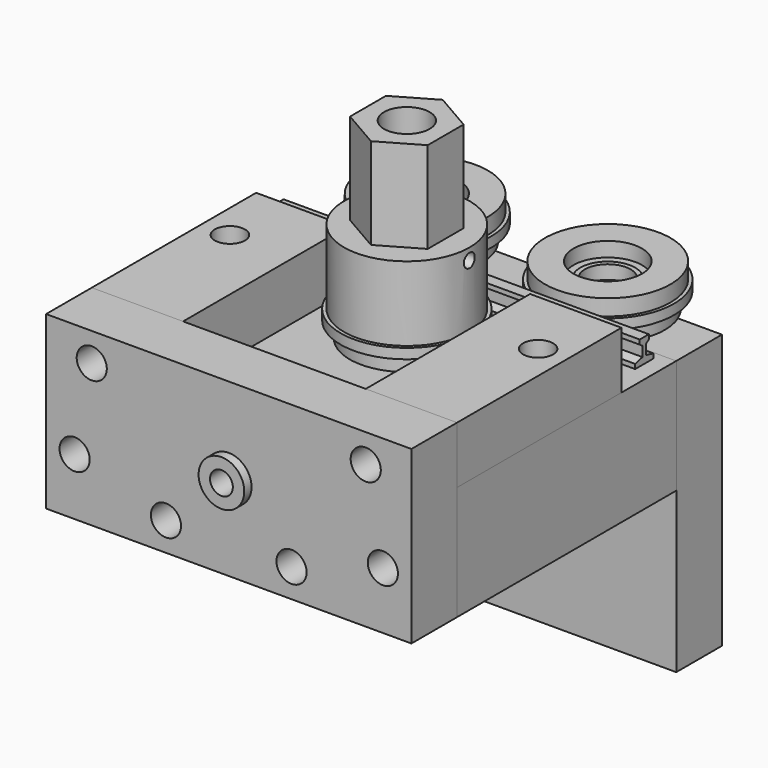
from build123d import *

# Parameters (mm, degrees)
F2_W           = 80
F2_H           = 12.5
F3_DEPTH       = 60
F6_DEPTH       = 40
F6_DEPTH_BACK  = 40
F4_W           = 2.5
F4_H           = 4
F12_R          = 7.5
F12_R_2        = 5
F13_DEPTH      = 20
F14_DEPTH      = 5
F17_R          = 3.3
F17_R_2        = 2.5
F18_DEPTH      = 60
F17_W          = 55
F17_H          = 12.5
F19_DEPTH      = 60
F21_DEPTH      = 12.5
F22_W          = 20
F22_H          = 45
F23_DEPTH      = 12.5
F24_W          = 80
F24_H          = 37.5
F25_DEPTH      = 12.5
F26_R          = 2.5
F27_DEPTH      = 25
F26_R_2        = 5
F26_R_3        = 3.3
F28_DEPTH      = 12.501
F29_R          = 2.5
F30_DEPTH      = 25
F29_R_2        = 3.3
F31_DEPTH      = 43.001
F32_DEPTH      = 20.751
F33_DEPTH      = 25
F34_R          = 4
F35_DEPTH      = 10
F37_DEPTH      = 14.5
F26_R_4        = 6
F38_DEPTH      = 2
F39_R          = 5
F39_R_2        = 2.5
F40_DEPTH      = 2
F41_DEPTH      = 2
F39_R_3        = 3.15
F42_DEPTH      = 2
F43_DEPTH      = 25
F44_DEPTH      = 60.001
F45_SIZE       = 2.7
F46_R          = 1
F47_DEPTH      = 3
F48_DEPTH      = 87.001
F49_R          = 1.5
F50_DEPTH      = 40.001
F50_DEPTH_BACK = 40.001


# Not quite as in the source:
# - a feature names something its author has since deleted; it is built from what else it names


with BuildPart() as f3:
    # F2 (on Top) → F3 (new body)
    with BuildSketch(Plane.XY):
        with Locations((0, 31.25)):
            Rectangle(F2_W, F2_H)
    extrude(amount=-F3_DEPTH)

    # F17 (on face) → F32 (cut, through all)
    with BuildSketch(Plane.XZ.offset(-25)):
        with Locations((-33.75, -6.25)):
            Circle(F17_R)
        with Locations((-33.75, -6.25)):
            Circle(F17_R_2, mode=Mode.SUBTRACT)
        with Locations((-33.75, -18.75)):
            Circle(F17_R)
        with Locations((-33.75, -18.75)):
            Circle(F17_R_2, mode=Mode.SUBTRACT)
        with Locations((-11.25, -18.75)):
            Circle(F17_R)
        with Locations((-11.25, -18.75)):
            Circle(F17_R_2, mode=Mode.SUBTRACT)
        with Locations((11.25, -18.75)):
            Circle(F17_R)
        with Locations((11.25, -18.75)):
            Circle(F17_R_2, mode=Mode.SUBTRACT)
        with Locations((33.75, -6.25)):
            Circle(F17_R)
        with Locations((33.75, -6.25)):
            Circle(F17_R_2, mode=Mode.SUBTRACT)
        with Locations((33.75, -18.75)):
            Circle(F17_R)
        with Locations((33.75, -18.75)):
            Circle(F17_R_2, mode=Mode.SUBTRACT)
        with Locations((-33.75, -6.25)):
            Circle(F17_R_2)
        with Locations((-33.75, -18.75)):
            Circle(F17_R_2)
        with Locations((-11.25, -18.75)):
            Circle(F17_R_2)
        with Locations((11.25, -18.75)):
            Circle(F17_R_2)
        with Locations((33.75, -6.25)):
            Circle(F17_R_2)
        with Locations((33.75, -18.75)):
            Circle(F17_R_2)
    extrude(amount=-F32_DEPTH, mode=Mode.SUBTRACT)

    # F39 (on face) → F40 (cut, through all)
    with BuildSketch(Plane.XY):
        with Locations((-20, 31.25)):
            Circle(F39_R)
        with Locations((-20, 31.25)):
            Circle(F39_R_2, mode=Mode.SUBTRACT)
    extrude(amount=-F40_DEPTH, mode=Mode.SUBTRACT)

    # F39 (on face) → F41 (cut, through all)
    with BuildSketch(Plane.XY):
        with Locations((20, 31.25)):
            Circle(F39_R)
        with Locations((20, 31.25)):
            Circle(F39_R_2, mode=Mode.SUBTRACT)
    extrude(amount=-F41_DEPTH, mode=Mode.SUBTRACT)

    # F39 (on face) → F43 (cut)
    with BuildSketch(Plane.XY):
        with Locations((20, 31.25)):
            Circle(F39_R_2)
        with Locations((-20, 31.25)):
            Circle(F39_R_2)
    extrude(amount=-F43_DEPTH, mode=Mode.SUBTRACT)


with BuildPart() as f5:
    # F4 (on Right) → F5 (revolve)
    with BuildSketch(Plane.YZ):
        Polygon((18.75, 4), (18.75, 3), (18.75, 1), (21.75, 1), (21.75, 2), (21.75, 7), (22.75, 7), (23.75, 7), (23.75, 10.2), (17.5, 10.2), (17.5, 8.2), (17.5, 7.2), (17.5, 6.7), (16.75, 6.7), (16.75, 4.5), (18.75, 4.5), align=None)
    revolve(axis=Axis((0, 31.25, 17.1989388764), (0, 0, -1)))


with BuildPart() as f6:
    # F4 (on Right) → F6 (new body, two sides)
    with BuildSketch(Plane.YZ) as f6_sk:
        Polygon((13.75, 4), (13.75, 3), (18.75, 3), (18.75, 4), (16.75, 4.5), (16.75, 6.7), (17.5, 7.2), (17.5, 8.2), (15, 8.2), (15, 7.2), (15.75, 6.7), (15.75, 4.5), align=None)
    extrude(amount=F6_DEPTH)
    extrude(f6_sk.sketch, amount=-F6_DEPTH_BACK)


with BuildPart() as f7:
    # F4 (on Right) → F7 (revolve)
    with BuildSketch(Plane.YZ):
        Polygon((25.25, 6.5), (25.25, 2.5), (25.25, 2), (26.25, 2), (26.25, 4), (26.25, 7), (25.25, 7), align=None)
        with Locations((24, 4.5)):
            Rectangle(F4_W, F4_H)
        Polygon((21.75, 7), (21.75, 2), (22.75, 2), (22.75, 2.5), (22.75, 6.5), (22.75, 7), align=None)
    revolve(axis=Axis((0, 31.25, 17.1989388764), (0, 0, -1)))


with BuildPart() as f8:
    # F4 (on Right) → F8 (revolve)
    with BuildSketch(Plane.YZ):
        Polygon((13.75, 1), (13.75, 3), (13.75, 4), (13.75, 4.5), (15.75, 4.5), (15.75, 6.7), (15, 6.7), (15, 7.2), (15, 8.2), (15, 23), (8.75, 23), (8.75, 15), (9.75, 15), (10.75, 15), (10.75, 10), (10.75, 7), (10.75, 2), (10.75, 1), align=None)
    revolve(axis=Axis((0, 1.25, 17.1989388764), (0, 0, -1)))


with BuildPart() as f9:
    # F4 (on Right) → F9 (revolve)
    with BuildSketch(Plane.YZ):
        Polygon((9.75, 2), (10.75, 2), (10.75, 7), (9.75, 7), (9.75, 6.5), (9.75, 2.5), align=None)
        with Locations((8.5, 4.5)):
            Rectangle(F4_W, F4_H)
        Polygon((7.25, 2), (7.25, 2.5), (7.25, 6.5), (7.25, 7), (6.25, 7), (6.25, 5), (6.25, 4), (6.25, 2), align=None)
    revolve(axis=Axis((0, 1.25, 17.1989388764), (0, 0, -1)))


with BuildPart() as f9b:
    # F4 (on Right) → F9, piece 2 (revolve)
    with BuildSketch(Plane.YZ):
        Polygon((7.25, 10), (7.25, 10.5), (7.25, 14.5), (7.25, 15), (6.25, 15), (6.25, 13), (6.25, 12), (6.25, 10), align=None)
        with Locations((8.5, 12.5)):
            Rectangle(F4_W, F4_H)
        Polygon((9.75, 10), (10.75, 10), (10.75, 15), (9.75, 15), (9.75, 14.5), (9.75, 10.5), align=None)
    revolve(axis=Axis((0, 1.25, 17.1989388764), (0, 0, -1)))


with BuildPart() as f10:
    # F4 (on Right) → F10 (revolve)
    with BuildSketch(Plane.YZ):
        Polygon((8.25, 2), (7.25, 2), (6.25, 2), (6.25, 4), (4.4, 4), (4.4, -2), (6.25, -2), (6.25, 0), (8.25, 0), align=None)
    revolve(axis=Axis((0, 1.25, 17.1989388764), (0, 0, -1)))


with BuildPart() as f10b:
    # F4 (on Right) → F10, piece 2 (revolve)
    with BuildSketch(Plane.YZ):
        Polygon((6.25, 7), (7.25, 7), (8.25, 7), (8.25, 10), (7.25, 10), (6.25, 10), (6.25, 12), (4.4, 12), (4.4, 5), (6.25, 5), align=None)
    revolve(axis=Axis((0, 1.25, 17.1989388764), (0, 0, -1)))


with BuildPart() as f10c:
    # F4 (on Right) → F10, piece 3 (revolve)
    with BuildSketch(Plane.YZ):
        Polygon((6.25, 15), (7.25, 15), (8.25, 15), (8.25, 17), (5.75, 17), (5.75, 27), (1.25, 27), (1.25, 22), (3.75, 22), (3.75, 17), (3.75, 13), (6.25, 13), align=None)
    revolve(axis=Axis((0, 1.25, 17.1989388764), (0, 0, -1)))

    # F46 (on face) → F47 (cut)
    with BuildSketch(Plane.XY.offset(27)):
        with Locations((-3, 1.25)):
            Circle(F46_R)
        with Locations((3, 1.25)):
            Circle(F46_R)
    extrude(amount=-F47_DEPTH, mode=Mode.SUBTRACT)

    # F46 (on face) → F48 (cut, through all)
    with BuildSketch(Plane.XY.offset(27)):
        with Locations((0, 1.25)):
            Circle(F46_R)
    extrude(amount=-F48_DEPTH, mode=Mode.SUBTRACT)


with BuildPart() as f11:
    # F4 (on Right) → F11 (revolve)
    with BuildSketch(Plane.YZ):
        Polygon((26.25, 2), (25.25, 2), (24.25, 2), (24.25, 0), (26.25, 0), (26.25, -2), (28.1, -2), (28.1, 4), (26.25, 4), align=None)
    revolve(axis=Axis((0, 31.25, 17.1989388764), (0, 0, -1)))


with BuildPart() as f13:
    # F12 (on face) → F13 (new body)
    with BuildSketch(Plane.XY.offset(23)):
        Polygon((0, 11.0649545762), (-8.5, 6.1574772881), (-8.5, -3.6574772881), (0, -8.5649545762), (8.5, -3.6574772881), (8.5, 6.1574772881), align=None)
        with Locations((0, 1.25)):
            Circle(F12_R, mode=Mode.SUBTRACT)
        with Locations((0, 1.25)):
            Circle(F12_R)
        with Locations((0, 1.25)):
            Circle(F12_R_2, mode=Mode.SUBTRACT)
    extrude(amount=F13_DEPTH)

    # F12 (on face) → F14 (join)
    with BuildSketch(Plane.XY.offset(23)):
        with Locations((0, 1.25)):
            Circle(F12_R)
        with Locations((0, 1.25)):
            Circle(F12_R_2, mode=Mode.SUBTRACT)
    extrude(amount=-F14_DEPTH)


with BuildPart() as f5_1:
    # F15: moved
    add(f5.part.moved(Location((20, 0, 0))))


with BuildPart() as f11_1:
    # F15: moved
    add(f11.part.moved(Location((20, 0, 0))))


with BuildPart() as f7_1:
    # F15: moved
    add(f7.part.moved(Location((20, 0, 0))))


with BuildPart() as f16_1:
    # F16: instance of F5
    add(f5_1.part.mirror(Plane.YZ))


with BuildPart() as f16_2:
    # F16: instance of F11
    add(f11_1.part.mirror(Plane.YZ))


with BuildPart() as f16_3:
    # F16: instance of F7
    add(f7_1.part.mirror(Plane.YZ))


with BuildPart() as f18:
    # F17 (on face) → F18 (new body)
    with BuildSketch(Plane.XZ.offset(-25)):
        Polygon((-27.5, 0), (-40, 0), (-40, -25), (-27.5, -25), (-27.5, -12.5), align=None)
        with Locations((-33.75, -18.75)):
            Circle(F17_R, mode=Mode.SUBTRACT)
        with Locations((-33.75, -6.25)):
            Circle(F17_R, mode=Mode.SUBTRACT)
        with Locations((-33.75, -18.75)):
            Circle(F17_R)
        with Locations((-33.75, -18.75)):
            Circle(F17_R_2, mode=Mode.SUBTRACT)
        with Locations((-33.75, -6.25)):
            Circle(F17_R)
        with Locations((-33.75, -6.25)):
            Circle(F17_R_2, mode=Mode.SUBTRACT)
        with Locations((-33.75, -18.75)):
            Circle(F17_R_2)
        with Locations((-33.75, -6.25)):
            Circle(F17_R_2)
    extrude(amount=F18_DEPTH)


with BuildPart() as f18b:
    # F17 (on face) → F18, piece 2 (new body)
    with BuildSketch(Plane.XZ.offset(-25)):
        Polygon((40, 0), (27.5, 0), (27.5, -12.5), (27.5, -25), (40, -25), align=None)
        with Locations((33.75, -18.75)):
            Circle(F17_R, mode=Mode.SUBTRACT)
        with Locations((33.75, -6.25)):
            Circle(F17_R, mode=Mode.SUBTRACT)
        with Locations((33.75, -18.75)):
            Circle(F17_R)
        with Locations((33.75, -18.75)):
            Circle(F17_R_2, mode=Mode.SUBTRACT)
        with Locations((33.75, -18.75)):
            Circle(F17_R_2)
        with Locations((33.75, -6.25)):
            Circle(F17_R)
        with Locations((33.75, -6.25)):
            Circle(F17_R_2, mode=Mode.SUBTRACT)
        with Locations((33.75, -6.25)):
            Circle(F17_R_2)
    extrude(amount=F18_DEPTH)


with BuildPart() as f19:
    # F17 (on face) → F19 (new body, through all)
    with BuildSketch(Plane.XZ.offset(-25)):
        with Locations((0, -18.75)):
            Rectangle(F17_W, F17_H)
        with Locations((-11.25, -18.75)):
            Circle(F17_R, mode=Mode.SUBTRACT)
        with Locations((11.25, -18.75)):
            Circle(F17_R, mode=Mode.SUBTRACT)
        with Locations((11.25, -18.75)):
            Circle(F17_R)
        with Locations((11.25, -18.75)):
            Circle(F17_R_2, mode=Mode.SUBTRACT)
        with Locations((-11.25, -18.75)):
            Circle(F17_R)
        with Locations((-11.25, -18.75)):
            Circle(F17_R_2, mode=Mode.SUBTRACT)
        with Locations((11.25, -18.75)):
            Circle(F17_R_2)
        with Locations((-11.25, -18.75)):
            Circle(F17_R_2)
    extrude(amount=F19_DEPTH)


with BuildPart() as f21:
    # F20 (on Top) → F21 (new body)
    with BuildSketch(Plane.XY):
        Polygon((-27.5, 18.25), (-27.5, -31.75), (-17.5, -31.75), (-9.9999999999, -23.75), (10.0000000001, -23.75), (17.5, -31.75), (27.5, -31.75), (27.5, 18.25), align=None)
    extrude(amount=-F21_DEPTH)


with BuildPart() as f23:
    # F22 (on face) → F23 (new body)
    with BuildSketch(Plane.XY):
        with Locations((-30, -12.5)):
            Rectangle(F22_W, F22_H)
    extrude(amount=F23_DEPTH)


with BuildPart() as f23b:
    # F22 (on face) → F23, piece 2 (new body)
    with BuildSketch(Plane.XY):
        with Locations((30, -12.5)):
            Rectangle(F22_W, F22_H)
    extrude(amount=F23_DEPTH)


with BuildPart() as f25:
    # F24 (on face) → F25 (new body)
    with BuildSketch(Plane.XZ.offset(35)):
        with Locations((0, -6.25)):
            Rectangle(F24_W, F24_H)
    extrude(amount=F25_DEPTH)

    # F26 (on face) → F28 (cut, through all)
    with BuildSketch(Plane(origin=(0, -35, 0), x_dir=(-1, 0, 0), z_dir=(0, 1, 0))):
        with Locations((-1e-10, -6.25)):
            Circle(F26_R_2)
        with Locations((-1e-10, -6.25)):
            Circle(F26_R, mode=Mode.SUBTRACT)
        with Locations((30, 6.25)):
            Circle(F26_R_3)
        with Locations((30, 6.25)):
            Circle(F26_R, mode=Mode.SUBTRACT)
        with Locations((33.75, -12.5)):
            Circle(F26_R_3)
        with Locations((33.75, -12.5)):
            Circle(F26_R, mode=Mode.SUBTRACT)
        with Locations((-33.75, -12.5)):
            Circle(F26_R_3)
        with Locations((-33.75, -12.5)):
            Circle(F26_R, mode=Mode.SUBTRACT)
        with Locations((-30, 6.25)):
            Circle(F26_R_3)
        with Locations((-30, 6.25)):
            Circle(F26_R, mode=Mode.SUBTRACT)
        with Locations((13.75, -18.75)):
            Circle(F26_R_3)
        with Locations((13.75, -18.75)):
            Circle(F26_R, mode=Mode.SUBTRACT)
        with Locations((-13.75, -18.75)):
            Circle(F26_R_3)
        with Locations((-13.75, -18.75)):
            Circle(F26_R, mode=Mode.SUBTRACT)
        with Locations((30, 6.25)):
            Circle(F26_R)
        with Locations((33.75, -12.5)):
            Circle(F26_R)
        with Locations((-33.75, -12.5)):
            Circle(F26_R)
        with Locations((-30, 6.25)):
            Circle(F26_R)
        with Locations((13.75, -18.75)):
            Circle(F26_R)
        with Locations((-13.75, -18.75)):
            Circle(F26_R)
        with Locations((-1e-10, -6.25)):
            Circle(F26_R)
    extrude(amount=-F28_DEPTH, mode=Mode.SUBTRACT)


with BuildPart() as f27_tool:
    # F26 (on face) → F27 (new body)
    with BuildSketch(Plane(origin=(0, -35, 0), x_dir=(-1, 0, 0), z_dir=(0, 1, 0))):
        with Locations((30, 6.25)):
            Circle(F26_R)
        with Locations((33.75, -12.5)):
            Circle(F26_R)
        with Locations((-33.75, -12.5)):
            Circle(F26_R)
        with Locations((-30, 6.25)):
            Circle(F26_R)
        with Locations((13.75, -18.75)):
            Circle(F26_R)
        with Locations((-13.75, -18.75)):
            Circle(F26_R)
    extrude(amount=F27_DEPTH)


with BuildPart() as f18_1:
    add(f18.part)

    # F27: cut by f27_tool
    add(f27_tool.part, mode=Mode.SUBTRACT)


with BuildPart() as f18b_1:
    add(f18b.part)

    # F27: cut by f27_tool
    add(f27_tool.part, mode=Mode.SUBTRACT)


with BuildPart() as f19_1:
    add(f19.part)

    # F27: cut by f27_tool
    add(f27_tool.part, mode=Mode.SUBTRACT)


with BuildPart() as f23_1:
    add(f23.part)

    # F27: cut by f27_tool
    add(f27_tool.part, mode=Mode.SUBTRACT)


with BuildPart() as f23b_1:
    add(f23b.part)

    # F27: cut by f27_tool
    add(f27_tool.part, mode=Mode.SUBTRACT)


with BuildPart() as f30_tool:
    # F29 (on face) → F30 (new body)
    with BuildSketch(Plane.XY):
        with Locations((-33.75, -5)):
            Circle(F29_R)
        with Locations((33.75, -5)):
            Circle(F29_R)
    extrude(amount=-F30_DEPTH)


with BuildPart() as f18_2:
    add(f18_1.part)

    # F30: cut by f30_tool
    add(f30_tool.part, mode=Mode.SUBTRACT)


with BuildPart() as f18b_2:
    add(f18b_1.part)

    # F30: cut by f30_tool
    add(f30_tool.part, mode=Mode.SUBTRACT)


with BuildPart() as f31_tool:
    # F29 (on face) → F31 (new body, through all)
    with BuildSketch(Plane.XY):
        with Locations((-33.75, -5)):
            Circle(F29_R_2)
        with Locations((-33.75, -5)):
            Circle(F29_R, mode=Mode.SUBTRACT)
        with Locations((33.75, -5)):
            Circle(F29_R_2)
        with Locations((33.75, -5)):
            Circle(F29_R, mode=Mode.SUBTRACT)
        with Locations((-33.75, -5)):
            Circle(F29_R)
        with Locations((33.75, -5)):
            Circle(F29_R)
    extrude(amount=F31_DEPTH)


with BuildPart() as f23_2:
    add(f23_1.part)

    # F31: cut by f31_tool
    add(f31_tool.part, mode=Mode.SUBTRACT)


with BuildPart() as f23b_2:
    add(f23b_1.part)

    # F31: cut by f31_tool
    add(f31_tool.part, mode=Mode.SUBTRACT)


with BuildPart() as f33_tool:
    # F17 (on face) → F33 (new body)
    with BuildSketch(Plane.XZ.offset(-25)):
        with Locations((-11.25, -18.75)):
            Circle(F17_R_2)
        with Locations((-33.75, -18.75)):
            Circle(F17_R_2)
        with Locations((-33.75, -6.25)):
            Circle(F17_R_2)
        with Locations((11.25, -18.75)):
            Circle(F17_R_2)
        with Locations((33.75, -18.75)):
            Circle(F17_R_2)
        with Locations((33.75, -6.25)):
            Circle(F17_R_2)
    extrude(amount=F33_DEPTH)


with BuildPart() as f18_3:
    add(f18_2.part)

    # F33: cut by f33_tool
    add(f33_tool.part, mode=Mode.SUBTRACT)


with BuildPart() as f18b_3:
    add(f18b_2.part)

    # F33: cut by f33_tool
    add(f33_tool.part, mode=Mode.SUBTRACT)


with BuildPart() as f19_2:
    add(f19_1.part)

    # F33: cut by f33_tool
    add(f33_tool.part, mode=Mode.SUBTRACT)


with BuildPart() as f35:
    # F34 (on face) → F35 (new body)
    with BuildSketch(Plane.XZ.offset(23.75)):
        with Locations((1e-10, -6.25)):
            Circle(F34_R)
    extrude(amount=-F35_DEPTH)


with BuildPart() as f21_1:
    add(f21.part)

    # F36: cut F35
    add(f35.part, mode=Mode.SUBTRACT)

    # F39 (on face) → F42 (cut, through all)
    with BuildSketch(Plane.XY):
        with Locations((0, 1.25)):
            Circle(F39_R)
        with Locations((0, 1.25)):
            Circle(F39_R_3, mode=Mode.SUBTRACT)
    extrude(amount=-F42_DEPTH, mode=Mode.SUBTRACT)

    # F39 (on face) → F44 (cut, through all)
    with BuildSketch(Plane.XY):
        with Locations((0, 1.25)):
            Circle(F39_R_3)
    extrude(amount=-F44_DEPTH, mode=Mode.SUBTRACT)

    # F45
    f45_edges = [f21_1.edges().sort_by_distance(p)[0] for p in [
        (-3.15, 1.25, -12.5),
    ]]
    chamfer(f45_edges, length=F45_SIZE)


with BuildPart() as f37:
    # F26 (on face) → F37 (new body)
    with BuildSketch(Plane(origin=(0, -35, 0), x_dir=(-1, 0, 0), z_dir=(0, 1, 0))):
        with Locations((-1e-10, -6.25)):
            Circle(F26_R_2)
        with Locations((-1e-10, -6.25)):
            Circle(F26_R, mode=Mode.SUBTRACT)
    extrude(amount=-F37_DEPTH)

    # F26 (on face) → F38 (join)
    with BuildSketch(Plane(origin=(0, -35, 0), x_dir=(-1, 0, 0), z_dir=(0, 1, 0))):
        with Locations((-1e-10, -6.25)):
            Circle(F26_R_4)
        with Locations((-1e-10, -6.25)):
            Circle(F26_R_2, mode=Mode.SUBTRACT)
        with Locations((-1e-10, -6.25)):
            Circle(F26_R_2)
        with Locations((-1e-10, -6.25)):
            Circle(F26_R, mode=Mode.SUBTRACT)
    extrude(amount=F38_DEPTH)


with BuildPart() as f50_tool:
    # F49 (on Right) → F50 (new body, two sides)
    with BuildSketch(Plane.YZ) as f50_sk:
        with Locations((1.25, 20.5)):
            Circle(F49_R)
    extrude(amount=-F50_DEPTH)
    extrude(f50_sk.sketch, amount=F50_DEPTH_BACK)


with BuildPart() as f8_1:
    add(f8.part)

    # F50: cut by f50_tool
    add(f50_tool.part, mode=Mode.SUBTRACT)


with BuildPart() as f13_1:
    add(f13.part)

    # F50: cut by f50_tool
    add(f50_tool.part, mode=Mode.SUBTRACT)


solid = Compound([f3.part, f6.part, f9.part, f9b.part, f10.part, f10b.part, f10c.part, f5_1.part, f11_1.part, f7_1.part, f16_1.part, f16_2.part, f16_3.part, f25.part, f23_2.part, f23b_2.part, f18_3.part, f18b_3.part, f19_2.part, f35.part, f21_1.part, f37.part, f8_1.part, f13_1.part])
